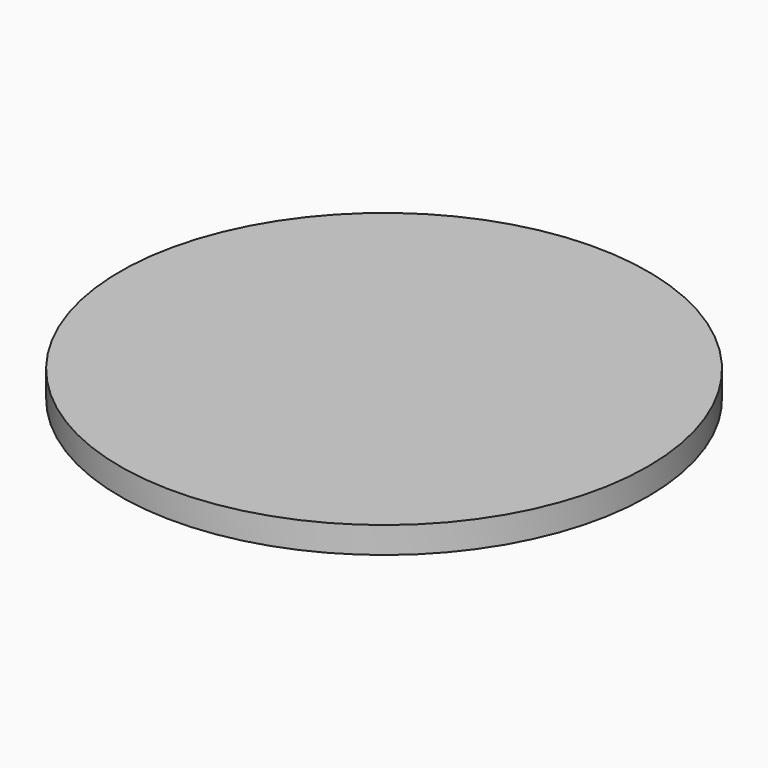
from build123d import *

# Parameters (mm, degrees)
F0_R     = 38.1
F1_DEPTH = 3.81


# Not quite as in the source:
# - a feature names something its author has since deleted; it is built from what else it names


with BuildPart() as f1:
    # F0 (on Top) → F1 (new body)
    with BuildSketch(Plane.XY):
        Circle(F0_R)
    extrude(amount=F1_DEPTH)


solid = f1.part
